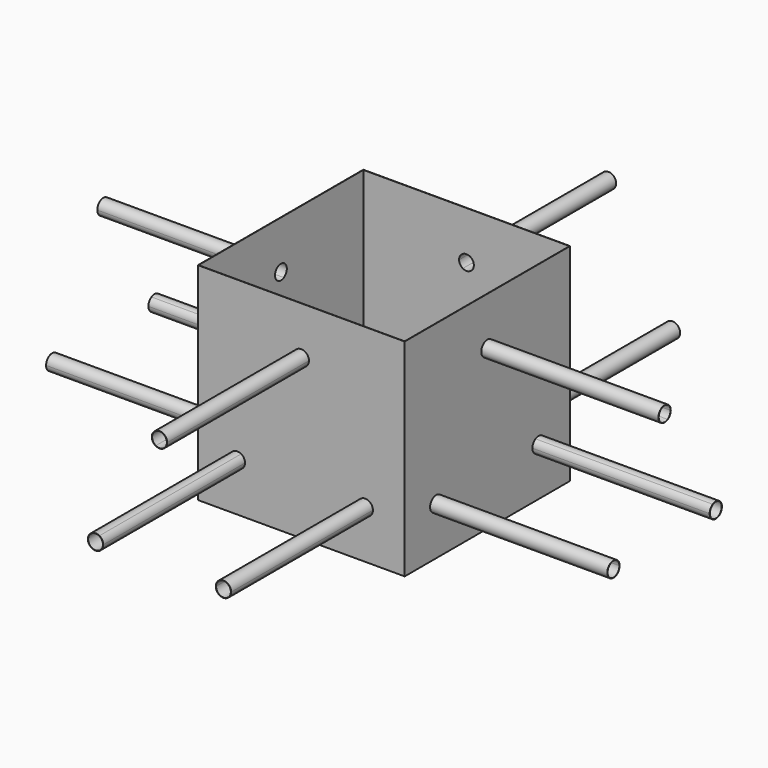
from build123d import *

# Parameters (mm, degrees)
F0_W      = 700
F0_H      = 700
F0_W_2    = 698
F0_H_2    = 698
F1_DEPTH  = 700
F6_DEPTH  = 600
F7_DEPTH  = 600
F8_DEPTH  = 600
F9_DEPTH  = 600
F10_DEPTH = 25
F11_DEPTH = 25
F12_DEPTH = 25
F13_DEPTH = 25
F14_DEPTH = 25
F15_DEPTH = 25
F16_DEPTH = 4990
F17_DEPTH = 4980


with BuildPart() as f1:
    # F0 (on Top) → F1 (new body)
    with BuildSketch(Plane.XY):
        Rectangle(F0_W, F0_H)
        Rectangle(F0_W_2, F0_H_2, mode=Mode.SUBTRACT)
    extrude(amount=-F1_DEPTH)

    # F2 (on face) → F6 (join)
    with BuildSketch(Plane.YZ.offset(350)):
        with BuildLine():
            ThreePointArc((25, -162.5), (21.650635, -175), (12.5, -184.150635))
            Line((12.5, -184.150635), (13, -185.01666))
            ThreePointArc((13, -185.01666), (22.51666, -175.5), (26, -162.5))
            ThreePointArc((26, -162.5), (-13, -139.98334), (-13, -185.01666))
            Line((-13, -185.01666), (-12.5, -184.150635))
            ThreePointArc((-12.5, -184.150635), (-12.5, -140.849365), (25, -162.5))
        make_face()
        with BuildLine():
            ThreePointArc((242.506351, -537.5), (229.506351, -514.98334), (203.506351, -514.98334))
            Line((203.506351, -514.98334), (204.006351, -515.849365))
            ThreePointArc((204.006351, -515.849365), (229.006351, -515.849365), (241.506351, -537.5))
            ThreePointArc((241.506351, -537.5), (216.506351, -562.5), (191.506351, -537.5))
            Line((191.506351, -537.5), (190.506351, -537.5))
            ThreePointArc((190.506351, -537.5), (216.506351, -563.5), (242.506351, -537.5))
        make_face()
        with BuildLine():
            Line((204.006351, -515.849365), (203.506351, -514.98334))
            ThreePointArc((203.506351, -514.98334), (193.98969, -524.5), (190.506351, -537.5))
            Line((190.506351, -537.5), (191.506351, -537.5))
            ThreePointArc((191.506351, -537.5), (194.855716, -525), (204.006351, -515.849365))
        make_face()
        with BuildLine():
            Line((13, -185.01666), (12.5, -184.150635))
            ThreePointArc((12.5, -184.150635), (0, -187.5), (-12.5, -184.150635))
            Line((-12.5, -184.150635), (-13, -185.01666))
            ThreePointArc((-13, -185.01666), (0, -188.5), (13, -185.01666))
        make_face()
        with BuildLine():
            Line((-204.006351, -515.849365), (-203.506351, -514.98334))
            ThreePointArc((-203.506351, -514.98334), (-239.023011, -550.5), (-190.506351, -537.5))
            Line((-190.506351, -537.5), (-191.506351, -537.5))
            ThreePointArc((-191.506351, -537.5), (-238.156986, -550), (-204.006351, -515.849365))
        make_face()
        with BuildLine():
            ThreePointArc((-190.506351, -537.5), (-193.98969, -524.5), (-203.506351, -514.98334))
            Line((-203.506351, -514.98334), (-204.006351, -515.849365))
            ThreePointArc((-204.006351, -515.849365), (-194.855716, -525), (-191.506351, -537.5))
            Line((-191.506351, -537.5), (-190.506351, -537.5))
        make_face()
    extrude(amount=F6_DEPTH)

    # F3 (on face) → F7 (join)
    with BuildSketch(Plane.XZ.offset(350)):
        with BuildLine():
            Line((13, -185.01666), (12.5, -184.150635))
            ThreePointArc((12.5, -184.150635), (0, -187.5), (-12.5, -184.150635))
            Line((-12.5, -184.150635), (-13, -185.01666))
            ThreePointArc((-13, -185.01666), (0, -188.5), (13, -185.01666))
        make_face()
        with BuildLine():
            ThreePointArc((25, -162.5), (21.650635, -175), (12.5, -184.150635))
            Line((12.5, -184.150635), (13, -185.01666))
            ThreePointArc((13, -185.01666), (22.51666, -175.5), (26, -162.5))
            ThreePointArc((26, -162.5), (-13, -139.98334), (-13, -185.01666))
            Line((-13, -185.01666), (-12.5, -184.150635))
            ThreePointArc((-12.5, -184.150635), (-12.5, -140.849365), (25, -162.5))
        make_face()
        with BuildLine():
            Line((-204.006351, -515.849365), (-203.506351, -514.98334))
            ThreePointArc((-203.506351, -514.98334), (-239.023011, -550.5), (-190.506351, -537.5))
            Line((-190.506351, -537.5), (-191.506351, -537.5))
            ThreePointArc((-191.506351, -537.5), (-238.156986, -550), (-204.006351, -515.849365))
        make_face()
        with BuildLine():
            ThreePointArc((-190.506351, -537.5), (-193.98969, -524.5), (-203.506351, -514.98334))
            Line((-203.506351, -514.98334), (-204.006351, -515.849365))
            ThreePointArc((-204.006351, -515.849365), (-194.855716, -525), (-191.506351, -537.5))
            Line((-191.506351, -537.5), (-190.506351, -537.5))
        make_face()
        with BuildLine():
            ThreePointArc((242.506351, -537.5), (229.506351, -514.98334), (203.506351, -514.98334))
            Line((203.506351, -514.98334), (204.006351, -515.849365))
            ThreePointArc((204.006351, -515.849365), (229.006351, -515.849365), (241.506351, -537.5))
            ThreePointArc((241.506351, -537.5), (216.506351, -562.5), (191.506351, -537.5))
            Line((191.506351, -537.5), (190.506351, -537.5))
            ThreePointArc((190.506351, -537.5), (216.506351, -563.5), (242.506351, -537.5))
        make_face()
        with BuildLine():
            Line((204.006351, -515.849365), (203.506351, -514.98334))
            ThreePointArc((203.506351, -514.98334), (193.98969, -524.5), (190.506351, -537.5))
            Line((190.506351, -537.5), (191.506351, -537.5))
            ThreePointArc((191.506351, -537.5), (194.855716, -525), (204.006351, -515.849365))
        make_face()
    extrude(amount=F7_DEPTH)

    # F4 (on face) → F8 (join)
    with BuildSketch(Plane(origin=(-350, 0, 0), x_dir=(0, -1, 0), z_dir=(-1, 0, 0))):
        with BuildLine():
            ThreePointArc((25, -162.5), (21.650635, -175), (12.5, -184.150635))
            Line((12.5, -184.150635), (13, -185.01666))
            ThreePointArc((13, -185.01666), (22.51666, -175.5), (26, -162.5))
            ThreePointArc((26, -162.5), (-13, -139.98334), (-13, -185.01666))
            Line((-13, -185.01666), (-12.5, -184.150635))
            ThreePointArc((-12.5, -184.150635), (-12.5, -140.849365), (25, -162.5))
        make_face()
        with BuildLine():
            Line((13, -185.01666), (12.5, -184.150635))
            ThreePointArc((12.5, -184.150635), (0, -187.5), (-12.5, -184.150635))
            Line((-12.5, -184.150635), (-13, -185.01666))
            ThreePointArc((-13, -185.01666), (0, -188.5), (13, -185.01666))
        make_face()
        with BuildLine():
            ThreePointArc((242.506351, -537.5), (229.506351, -514.98334), (203.506351, -514.98334))
            Line((203.506351, -514.98334), (204.006351, -515.849365))
            ThreePointArc((204.006351, -515.849365), (229.006351, -515.849365), (241.506351, -537.5))
            ThreePointArc((241.506351, -537.5), (216.506351, -562.5), (191.506351, -537.5))
            Line((191.506351, -537.5), (190.506351, -537.5))
            ThreePointArc((190.506351, -537.5), (216.506351, -563.5), (242.506351, -537.5))
        make_face()
        with BuildLine():
            Line((204.006351, -515.849365), (203.506351, -514.98334))
            ThreePointArc((203.506351, -514.98334), (193.98969, -524.5), (190.506351, -537.5))
            Line((190.506351, -537.5), (191.506351, -537.5))
            ThreePointArc((191.506351, -537.5), (194.855716, -525), (204.006351, -515.849365))
        make_face()
        with BuildLine():
            Line((-204.006351, -515.849365), (-203.506351, -514.98334))
            ThreePointArc((-203.506351, -514.98334), (-239.023011, -550.5), (-190.506351, -537.5))
            Line((-190.506351, -537.5), (-191.506351, -537.5))
            ThreePointArc((-191.506351, -537.5), (-238.156986, -550), (-204.006351, -515.849365))
        make_face()
        with BuildLine():
            ThreePointArc((-190.506351, -537.5), (-193.98969, -524.5), (-203.506351, -514.98334))
            Line((-203.506351, -514.98334), (-204.006351, -515.849365))
            ThreePointArc((-204.006351, -515.849365), (-194.855716, -525), (-191.506351, -537.5))
            Line((-191.506351, -537.5), (-190.506351, -537.5))
        make_face()
    extrude(amount=F8_DEPTH)

    # F5 (on face) → F9 (join)
    with BuildSketch(Plane(origin=(0, 350, 0), x_dir=(-1, 0, 0), z_dir=(0, 1, 0))):
        with BuildLine():
            Line((13, -185.01666), (12.5, -184.150635))
            ThreePointArc((12.5, -184.150635), (0, -187.5), (-12.5, -184.150635))
            Line((-12.5, -184.150635), (-13, -185.01666))
            ThreePointArc((-13, -185.01666), (0, -188.5), (13, -185.01666))
        make_face()
        with BuildLine():
            ThreePointArc((25, -162.5), (21.650635, -175), (12.5, -184.150635))
            Line((12.5, -184.150635), (13, -185.01666))
            ThreePointArc((13, -185.01666), (22.51666, -175.5), (26, -162.5))
            ThreePointArc((26, -162.5), (-13, -139.98334), (-13, -185.01666))
            Line((-13, -185.01666), (-12.5, -184.150635))
            ThreePointArc((-12.5, -184.150635), (-12.5, -140.849365), (25, -162.5))
        make_face()
        with BuildLine():
            Line((-204.006351, -515.849365), (-203.506351, -514.98334))
            ThreePointArc((-203.506351, -514.98334), (-239.023011, -550.5), (-190.506351, -537.5))
            Line((-190.506351, -537.5), (-191.506351, -537.5))
            ThreePointArc((-191.506351, -537.5), (-238.156986, -550), (-204.006351, -515.849365))
        make_face()
        with BuildLine():
            ThreePointArc((-190.506351, -537.5), (-193.98969, -524.5), (-203.506351, -514.98334))
            Line((-203.506351, -514.98334), (-204.006351, -515.849365))
            ThreePointArc((-204.006351, -515.849365), (-194.855716, -525), (-191.506351, -537.5))
            Line((-191.506351, -537.5), (-190.506351, -537.5))
        make_face()
        with BuildLine():
            Line((204.006351, -515.849365), (203.506351, -514.98334))
            ThreePointArc((203.506351, -514.98334), (193.98969, -524.5), (190.506351, -537.5))
            Line((190.506351, -537.5), (191.506351, -537.5))
            ThreePointArc((191.506351, -537.5), (194.855716, -525), (204.006351, -515.849365))
        make_face()
        with BuildLine():
            ThreePointArc((242.506351, -537.5), (229.506351, -514.98334), (203.506351, -514.98334))
            Line((203.506351, -514.98334), (204.006351, -515.849365))
            ThreePointArc((204.006351, -515.849365), (229.006351, -515.849365), (241.506351, -537.5))
            ThreePointArc((241.506351, -537.5), (216.506351, -562.5), (191.506351, -537.5))
            Line((191.506351, -537.5), (190.506351, -537.5))
            ThreePointArc((190.506351, -537.5), (216.506351, -563.5), (242.506351, -537.5))
        make_face()
    extrude(amount=F9_DEPTH)

    # F10 (cut): a face of the model
    f10_faces = [f1.faces().sort_by_distance(p)[0] for p in [
        (350, -216.506351, -537.5),
    ]]
    extrude(f10_faces, amount=-F10_DEPTH, mode=Mode.SUBTRACT)

    # F11 (cut): a face of the model
    f11_faces = [f1.faces().sort_by_distance(p)[0] for p in [
        (350, 216.506351, -537.5),
    ]]
    extrude(f11_faces, amount=-F11_DEPTH, mode=Mode.SUBTRACT)

    # F12 (cut): a face of the model
    f12_faces = [f1.faces().sort_by_distance(p)[0] for p in [
        (-350, 216.506351, -537.5),
    ]]
    extrude(f12_faces, amount=-F12_DEPTH, mode=Mode.SUBTRACT)

    # F13 (cut): a face of the model
    f13_faces = [f1.faces().sort_by_distance(p)[0] for p in [
        (-350, -216.506351, -537.5),
    ]]
    extrude(f13_faces, amount=-F13_DEPTH, mode=Mode.SUBTRACT)

    # F14 (cut): faces of the model
    f14_faces = [f1.faces().sort_by_distance(p)[0] for p in [
        (-216.506351, 350, -537.5),
        (216.506351, 350, -537.5),
    ]]
    extrude(f14_faces, amount=-F14_DEPTH, mode=Mode.SUBTRACT)

    # F15 (cut): faces of the model
    f15_faces = [f1.faces().sort_by_distance(p)[0] for p in [
        (216.506351, -350, -537.5),
        (-216.506351, -350, -537.5),
    ]]
    extrude(f15_faces, amount=-F15_DEPTH, mode=Mode.SUBTRACT)

    # F16 (cut): a face of the model
    f16_faces = [f1.faces().sort_by_distance(p)[0] for p in [
        (350, 0, -162.5),
    ]]
    extrude(f16_faces, amount=-F16_DEPTH, mode=Mode.SUBTRACT)

    # F17 (cut): a face of the model
    f17_faces = [f1.faces().sort_by_distance(p)[0] for p in [
        (0, 350, -162.5),
    ]]
    extrude(f17_faces, amount=-F17_DEPTH, mode=Mode.SUBTRACT)


solid = f1.part
